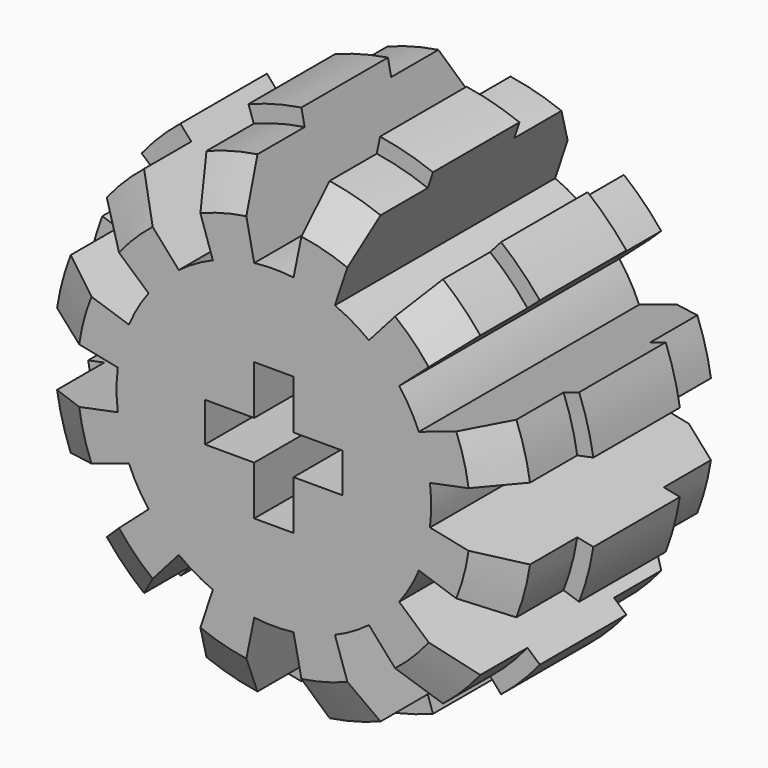
from build123d import *

# Parameters (mm, degrees)
F0_R            = 6.5
F1_DEPTH        = 7
F5_DEPTH        = 7.001
F5_COPIES_COUNT = 12


# Not quite as in the source:
# - a pattern or mirror of a feature is missing from the dataset's text; its kind, count and spacing are read off the source's solid


with BuildPart() as f1:
    # F0 (on Front) → F1 (new body)
    with BuildSketch(Plane.XZ):
        Circle(F0_R)
        Polygon((-1.75, 0.5), (-0.5, 0.5), (-0.5, 1.75), (0.5, 1.75), (0.5, 0.5), (1.75, 0.5), (1.75, -0.5), (0.5, -0.5), (0.5, -1.75), (-0.5, -1.75), (-0.5, -0.5), (-1.75, -0.5), align=None, mode=Mode.SUBTRACT)
    extrude(amount=F1_DEPTH)

    # F2 (on Right) → F3 (revolve, cut)
    with BuildSketch(Plane.YZ):
        Polygon((-7, 8), (-7, 5), (-6.375, 6.0825317547), (-4.875, 6.0825317547), (-4.875, 6.5), (-2.125, 6.5), (-2.125, 6.0825317547), (-0.625, 6.0825317547), (0, 5), (0, 8), align=None)
    revolve(axis=Axis((0, 2.603987056, 0), (0, 1, 0)), mode=Mode.SUBTRACT)

    # F4 (on Front) → F5 (cut, through all)
    with BuildSketch(Plane.XZ):
        with BuildLine():
            Line((0.5, 3.9686269666), (1, 6.4226162893))
            ThreePointArc((1, 6.4226162893), (0, 6.5), (-1, 6.4226162893))
            Line((-1, 6.4226162893), (-0.5, 3.9686269666))
            ThreePointArc((-0.5, 3.9686269666), (0, 4), (0.5, 3.9686269666))
        make_face()
    f5 = extrude(amount=F5_DEPTH, mode=Mode.SUBTRACT)

    # F5_copies: F5 ×12 about axis
    f5_copies_axis = Axis((0, 0, 0), (0, 1, 0))
    for i in range(1, F5_COPIES_COUNT):
        add(f5.rotate(f5_copies_axis, i * 360 / F5_COPIES_COUNT), mode=Mode.SUBTRACT)


solid = f1.part
